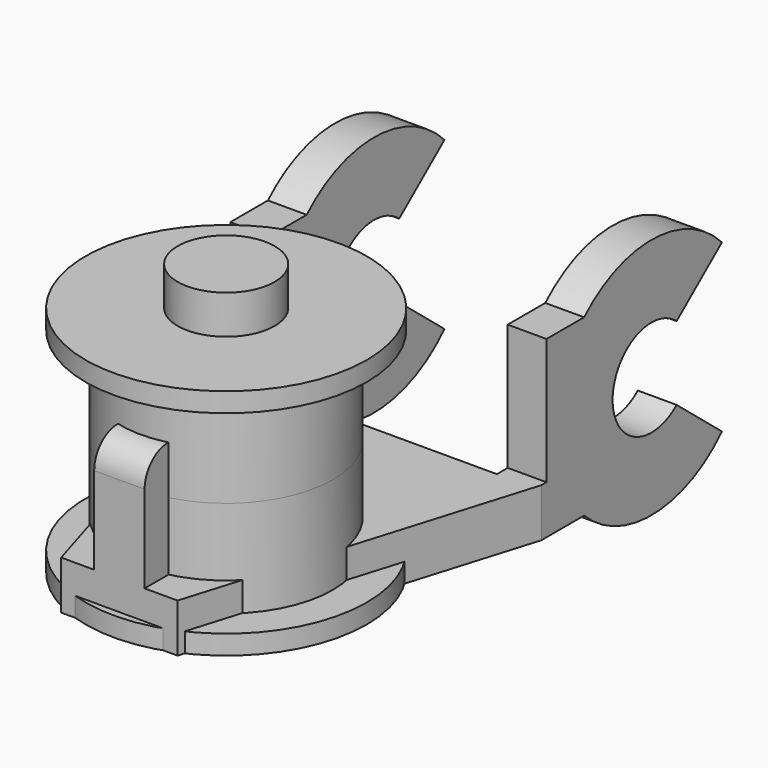
from build123d import *

# Parameters (mm, degrees)
F0_R           = 7.25
F1_DEPTH       = 1
F2_R           = 5.5
F3_DEPTH       = 5
F4_R           = 2.5
F5_DEPTH       = 2
F8_DEPTH       = 9
F10_DEPTH      = 8.15
F10_DEPTH_BACK = 8.15
F11_W          = 12.3
F11_H          = 13.3198345661
F12_DEPTH      = 25
F12_DEPTH_BACK = 25
F13_W          = 18.4948361841
F13_H          = 7.169587491
F14_DEPTH      = 25
F14_DEPTH_BACK = 25
F16_DEPTH      = 1.3
F16_DEPTH_BACK = 1.3
F17_R          = 1.5


with BuildPart() as f1:
    # F0 (on Top) → F1 (new body)
    with BuildSketch(Plane.XY):
        Circle(F0_R)
    extrude(amount=F1_DEPTH)

    # F2 (on face) → F3 (join)
    with BuildSketch(Plane.XY.offset(1)):
        Circle(F2_R)
    extrude(amount=F3_DEPTH)

    # F4 (on face) → F5 (join)
    with BuildSketch(Plane(origin=(0, 0, 0), x_dir=(1, 0, 0), z_dir=(0, 0, -1))):
        Circle(F4_R)
    extrude(amount=F5_DEPTH)

    # F6: F1 across face


with BuildPart() as f1_1:
    add(f1.part)
    add(f1.part.mirror(Plane.XY.offset(6)))


with BuildPart() as f8:
    # F7 (on Top) → F8 (new body)
    with BuildSketch(Plane.XY):
        Polygon((8.15, 13.1216109544), (0, 13.1216109544), (-8.15, 13.1216109544), (-8.15, 10.1216109544), (-3, -6.8783890456), (0, -6.8783890456), (3, -6.8783890456), (8.15, 10.1216109544), align=None)
    extrude(amount=F8_DEPTH)

    # F9 (on Right) → F10 (join, two sides)
    with BuildSketch(Plane.YZ) as f10_sk:
        with BuildLine():
            Line((18.8368415974, 6.399459286), (21.7546150774, 8.792052357))
            ThreePointArc((21.7546150774, 8.792052357), (10.9614018351, 4.5), (21.7546150774, 0.207947643))
            Line((21.7546150774, 0.207947643), (18.8368415974, 2.600540714))
            ThreePointArc((18.8368415974, 2.600540714), (14.7114018351, 4.5), (18.8368415974, 6.399459286))
        make_face()
    extrude(amount=F10_DEPTH)
    extrude(f10_sk.sketch, amount=-F10_DEPTH_BACK)

    # F11 (on Top) → F12 (cut, two sides)
    with BuildSketch(Plane.XY) as f12_sk:
        with Locations((0, 16.4145323604)):
            Rectangle(F11_W, F11_H)
    extrude(amount=F12_DEPTH, mode=Mode.SUBTRACT)
    extrude(f12_sk.sketch, amount=-F12_DEPTH_BACK, mode=Mode.SUBTRACT)

    # F13 (on Right) → F14 (cut, two sides)
    with BuildSketch(Plane.YZ) as f14_sk:
        with Locations((1.2051223312, 6.0847937455)):
            Rectangle(F13_W, F13_H)
    extrude(amount=-F14_DEPTH, mode=Mode.SUBTRACT)
    extrude(f14_sk.sketch, amount=F14_DEPTH_BACK, mode=Mode.SUBTRACT)

    # F15 (on Right) → F16 (join, two sides)
    with BuildSketch(Plane.YZ) as f16_sk:
        with BuildLine():
            Line((-6.8783890456, 8.5), (-6.8783890456, 2.5))
            Line((-6.8783890456, 2.5), (2.1216109544, 2.5))
            Line((2.1216109544, 2.5), (2.1216109544, 8.5))
            Line((2.1216109544, 8.5), (-0.7507189293, 8.5))
            Line((-0.7507189293, 8.5), (-1.2240023592, 7.6332150435))
            ThreePointArc((-1.2240023592, 7.6332150435), (-2.3783890456, 4), (-3.532775732, 7.6332150435))
            Line((-3.532775732, 7.6332150435), (-4.0060591619, 8.5))
            Line((-4.0060591619, 8.5), (-6.8783890456, 8.5))
        make_face()
    extrude(amount=F16_DEPTH)
    extrude(f16_sk.sketch, amount=-F16_DEPTH_BACK)

    # F17
    f17_edges = [f8.edges().sort_by_distance(p)[0] for p in [
        (0, -6.878389, 8.5),
        (0, 2.121611, 8.5),
    ]]
    fillet(f17_edges, radius=F17_R)


solid = Compound([f1_1.part, f8.part])
